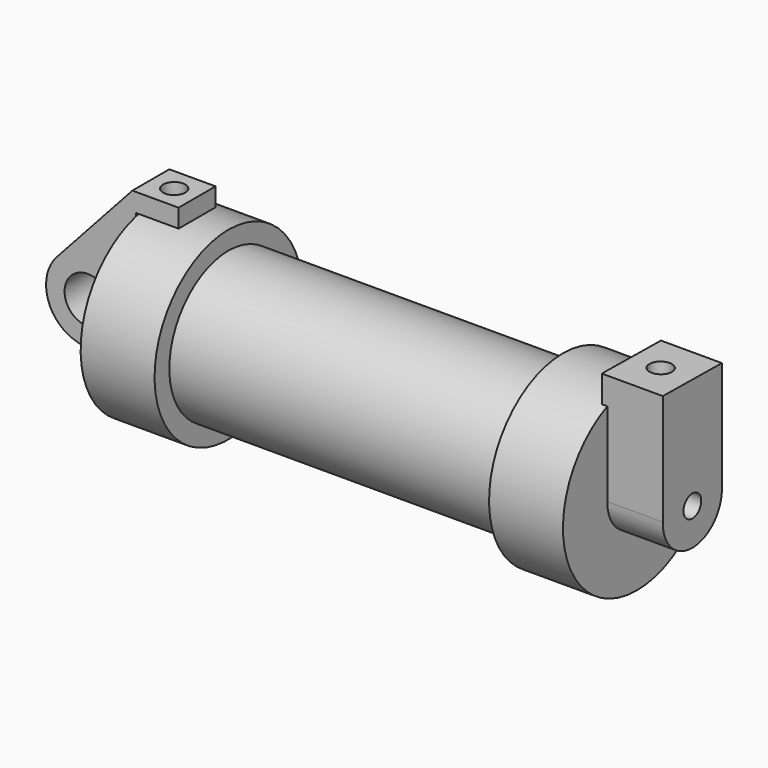
from build123d import *

# Parameters (mm, degrees)
F0_W          = 5.842
F0_H          = 12.7
F0_R          = 3.175
F2_DEPTH      = 3.175
F3_R          = 1.524
F4_DEPTH      = 7.62
F4_DEPTH_BACK = 0.762
F5_R          = 1.524
F6_DEPTH      = 17.78
F6_TAPER      = -3
F7_R          = 1.524
F8_DEPTH      = 10.414


# Not quite as in the source:
# - ends of sketch curves that miss each other by under 0.0002 mm in the source are joined


with BuildPart() as f1:
    # F0 (on Front) → F1 (revolve)
    with BuildSketch(Plane.XZ):
        Polygon((5.842, 12.7), (5.842, 0), (66.294, 0), (66.294, 12.7), (56.134, 12.7), (56.134, 10.16), (10.16, 10.16), (10.16, 12.7), align=None)
        with Locations((2.921, 6.35)):
            Rectangle(F0_W, F0_H)
    revolve(axis=Axis((33.147, 0, 0), (-1, 0, 0)))

    # F3 (on face) → F4 (join, two sides)
    with BuildSketch(Plane.YZ.offset(66.294)) as f4_sk:
        with BuildLine():
            ThreePointArc((5.0799454558, -0.0235407301), (5.0799863639, -0.0117703966), (5.08, 0))
            ThreePointArc((5.08, 0), (0.056082159, 5.0796904228), (-5.0787617289, 0.1121574827))
            ThreePointArc((-5.0787617289, 0.1121574827), (-0.0678516878, -5.0795468448), (5.0799454558, -0.0235407301))
        make_face()
        Circle(F3_R, mode=Mode.SUBTRACT)
        with BuildLine():
            ThreePointArc((-5.0787617289, 11.6402826126), (0.0006457603, 12.6999999836), (5.0799454558, 11.6397660701))
            Line((5.0799454558, 11.6397660701), (5.0799454558, 15.2164592699))
            Line((5.0799454558, 15.2164592699), (-5.0787617289, 15.3521574827))
            Line((-5.0787617289, 15.3521574827), (-5.0787617289, 11.6402826126))
        make_face()
        with BuildLine():
            ThreePointArc((-5.0787617289, 0.1121574827), (0.056082159, 5.0796904228), (5.08, 0))
            Line((5.08, 0), (5.0799454558, 11.6397660701))
            ThreePointArc((5.0799454558, 11.6397660701), (0.0006457603, 12.6999999836), (-5.0787617289, 11.6402826126))
            Line((-5.0787617289, 11.6402826126), (-5.0787617289, 0.1121574827))
        make_face()
    extrude(amount=F4_DEPTH)
    extrude(f4_sk.sketch, amount=-F4_DEPTH_BACK)

    # F7 (on face) → F8 (cut)
    with BuildSketch(Plane(origin=(0, 0.2041287691, 15.2815895663), x_dir=(1, 0, 0), z_dir=(0, 0.0133566315, 0.9999107962))):
        with Locations((69.5667713881, -0.2035550635)):
            Circle(F7_R)
    extrude(amount=-F8_DEPTH, mode=Mode.SUBTRACT)


with BuildPart() as f2:
    # F0 (on Front) → F2 (new body, symmetric)
    with BuildSketch(Plane.XZ):
        with BuildLine():
            Line((-0.9398, 0), (0, 0))
            Line((0, 0), (0, 12.7))
            Line((0, 12.7), (5.842, 12.7))
            Line((5.842, 12.7), (5.842, 15.24))
            Line((5.842, 15.24), (-0.508, 15.24))
            Line((-0.508, 15.24), (-10.8806298187, 3.8475430269))
            ThreePointArc((-10.8806298187, 3.8475430269), (-4.5919612295, 5.3297205562), (-0.9398, 0))
        make_face()
        with BuildLine():
            Line((5.842, 0), (0, 0))
            Line((0, 0), (-0.9398, 0))
            ThreePointArc((-0.9398, 0), (-3.1957909266, -4.5493385486), (-8.1826630726, -5.5069827884))
            Line((-8.1826630726, -5.5069827884), (5.842, -9.398))
            Line((5.842, -9.398), (5.842, 0))
        make_face()
        with BuildLine():
            ThreePointArc((-8.1826630726, -5.5069827884), (-3.1957909266, -4.5493385486), (-0.9398, 0))
            ThreePointArc((-0.9398, 0), (-4.5919612295, 5.3297205562), (-10.8806298187, 3.8475430269))
            ThreePointArc((-10.8806298187, 3.8475430269), (-12.1459778134, -1.5837270034), (-8.1826630726, -5.5069827884))
        make_face()
        with Locations((-6.6548, 0)):
            Circle(F0_R, mode=Mode.SUBTRACT)
    extrude(amount=F2_DEPTH, both=True)

    # F5 (on face) → F6 (cut)
    with BuildSketch(Plane.XY.offset(15.24)):
        with Locations((2.6962365955, 0)):
            Circle(F5_R)
    extrude(amount=-F6_DEPTH, taper=F6_TAPER, mode=Mode.SUBTRACT)


solid = Compound([f1.part, f2.part])
